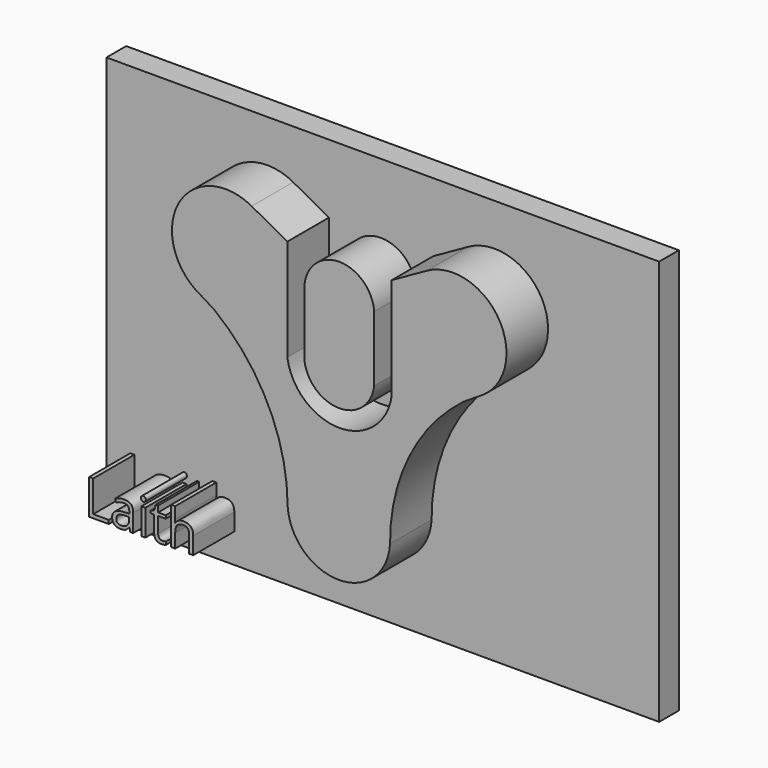
from build123d import *

# Parameters (mm, degrees)
F1_DEPTH     = 15.39817
F0_W         = 163.8866513968
F0_H         = 120.1637163758
F2_DEPTH     = 7.30042
F3_TEXT_SIZE = 14.5802326086
F4_DEPTH     = 15.24


# Not quite as in the source:
# - Text() gives the source's letters only with a copy of the font that has no kerning and outlines rounded to 1/6400 em; it was checked with that copy


with BuildPart() as f1:
    # F0 (on Front) → F1 (new body)
    with BuildSketch(Plane.XZ):
        with BuildLine():
            Line((25.2868216485, 45.5188639462), (14.9562442675, 39.715051651))
            Line((14.9562442675, 39.715051651), (14.9562442675, 9.5035806298))
            ThreePointArc((14.9562442675, 9.5035806298), (-0.5198442377, -3.9046924703), (-15.995932743, 9.5035806298))
            Line((-15.995932743, 9.5035806298), (-15.995932743, 39.715051651))
            Line((-15.995932743, 39.715051651), (-26.5831723809, 45.5188639462))
            ThreePointArc((-26.5831723809, 45.5188639462), (-47.8560530267, 39.8727264749), (-43.2591997087, 18.3487106115))
            Line((-43.2591997087, 18.3487106115), (-37.7070344985, 14.9252964184))
            ThreePointArc((-37.7070344985, 14.9252964184), (-21.6988985987, -4.6496789904), (-15.8998668194, -29.262913391))
            ThreePointArc((-15.8998668194, -29.262913391), (-0.7185637951, -43.6390577842), (14.4627392292, -29.262913391))
            ThreePointArc((14.4627392292, -29.262913391), (20.148592377, -4.5950626204), (36.2665131688, 14.9252964184))
            Line((36.2665131688, 14.9252964184), (41.6454896331, 18.3487106115))
            ThreePointArc((41.6454896331, 18.3487106115), (46.7179439882, 39.9124542781), (25.2868216485, 45.5188639462))
        make_face()
    extrude(amount=F1_DEPTH)


with BuildPart() as f1b:
    # F0 (on Front) → F1, piece 2 (new body)
    with BuildSketch(Plane.XZ):
        with BuildLine():
            ThreePointArc((9.7599746659, 29.8606865108), (-0.589103438, 39.4640683192), (-10.9381815419, 29.8606865108))
            Line((-10.9381815419, 29.8606865108), (-10.9381815419, 10.4503789917))
            ThreePointArc((-10.9381815419, 10.4503789917), (-0.589103438, 1.2185059392), (9.7599746659, 10.4503789917))
            Line((9.7599746659, 10.4503789917), (9.7599746659, 29.8606865108))
        make_face()
    extrude(amount=F1_DEPTH)


with BuildPart() as f2:
    # F0 (on Front) → F2 (new body)
    with BuildSketch(Plane.XZ):
        Rectangle(F0_W, F0_H)
        with BuildLine():
            Line((14.9562442675, 9.5035806298), (14.9562442675, 39.715051651))
            Line((14.9562442675, 39.715051651), (25.2868216485, 45.5188639462))
            ThreePointArc((25.2868216485, 45.5188639462), (46.7179439882, 39.9124542781), (41.6454896331, 18.3487106115))
            Line((41.6454896331, 18.3487106115), (36.2665131688, 14.9252964184))
            ThreePointArc((36.2665131688, 14.9252964184), (20.148592377, -4.5950626204), (14.4627392292, -29.262913391))
            ThreePointArc((14.4627392292, -29.262913391), (-0.7185637951, -43.6390577842), (-15.8998668194, -29.262913391))
            ThreePointArc((-15.8998668194, -29.262913391), (-21.6988985987, -4.6496789904), (-37.7070344985, 14.9252964184))
            Line((-37.7070344985, 14.9252964184), (-43.2591997087, 18.3487106115))
            ThreePointArc((-43.2591997087, 18.3487106115), (-47.8560530267, 39.8727264749), (-26.5831723809, 45.5188639462))
            Line((-26.5831723809, 45.5188639462), (-15.995932743, 39.715051651))
            Line((-15.995932743, 39.715051651), (-15.995932743, 9.5035806298))
            ThreePointArc((-15.995932743, 9.5035806298), (-0.5198442377, -3.9046924703), (14.9562442675, 9.5035806298))
        make_face(mode=Mode.SUBTRACT)
        with BuildLine():
            Line((-10.9381815419, 10.4503789917), (-10.9381815419, 29.8606865108))
            ThreePointArc((-10.9381815419, 29.8606865108), (-0.589103438, 39.4640683192), (9.7599746659, 29.8606865108))
            Line((9.7599746659, 29.8606865108), (9.7599746659, 10.4503789917))
            ThreePointArc((9.7599746659, 10.4503789917), (-0.589103438, 1.2185059392), (-10.9381815419, 10.4503789917))
        make_face(mode=Mode.SUBTRACT)
    extrude(amount=-F2_DEPTH)

    # F3 (on Front) → F4 (join)
    with BuildSketch(Plane.XZ):
        with Locations((-76.3215944171, -51.3539388776)):
            Text('Laith', F3_TEXT_SIZE, font='Open Sans', text_align=(TextAlign.LEFT, TextAlign.BOTTOM))
    extrude(amount=F4_DEPTH)


solid = Compound([f1.part, f1b.part, f2.part])
